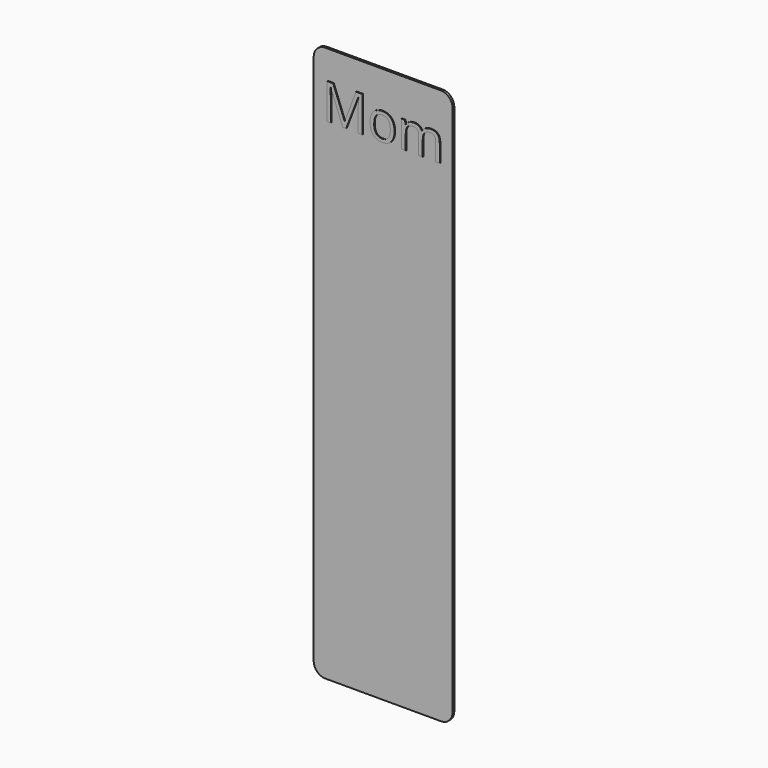
from build123d import *

# Parameters (mm, degrees)
F1_DEPTH     = 0.6
F2_TEXT_SIZE = 13.7080618373
F3_DEPTH     = 0.2


# Not quite as in the source:
# - Text() gives the source's letters only with a copy of the font that has no kerning and outlines rounded to 1/6400 em; it was checked with that copy


with BuildPart() as f1:
    # F0 (on Front) → F1 (new body)
    with BuildSketch(Plane.XZ):
        with BuildLine():
            Line((34.925, 0), (3.175, 0))
            ThreePointArc((3.175, 0), (0.9299359697, -0.9299359697), (0, -3.175))
            Line((0, -3.175), (0, -149.225))
            ThreePointArc((0, -149.225), (0.9299359697, -151.4700640303), (3.175, -152.4))
            Line((3.175, -152.4), (34.925, -152.4))
            ThreePointArc((34.925, -152.4), (37.1700640303, -151.4700640303), (38.1, -149.225))
            Line((38.1, -149.225), (38.1, -3.175))
            ThreePointArc((38.1, -3.175), (37.1700640303, -0.9299359697), (34.925, 0))
        make_face()
    extrude(amount=F1_DEPTH)

    # F2 (on face) → F3 (join)
    with BuildSketch(Plane.XZ.offset(0.6)):
        with Locations((2.4578904653, -17.5504772647)):
            Text('Mom', F2_TEXT_SIZE, font='Open Sans', text_align=(TextAlign.LEFT, TextAlign.BOTTOM))
    extrude(amount=F3_DEPTH)


solid = f1.part
